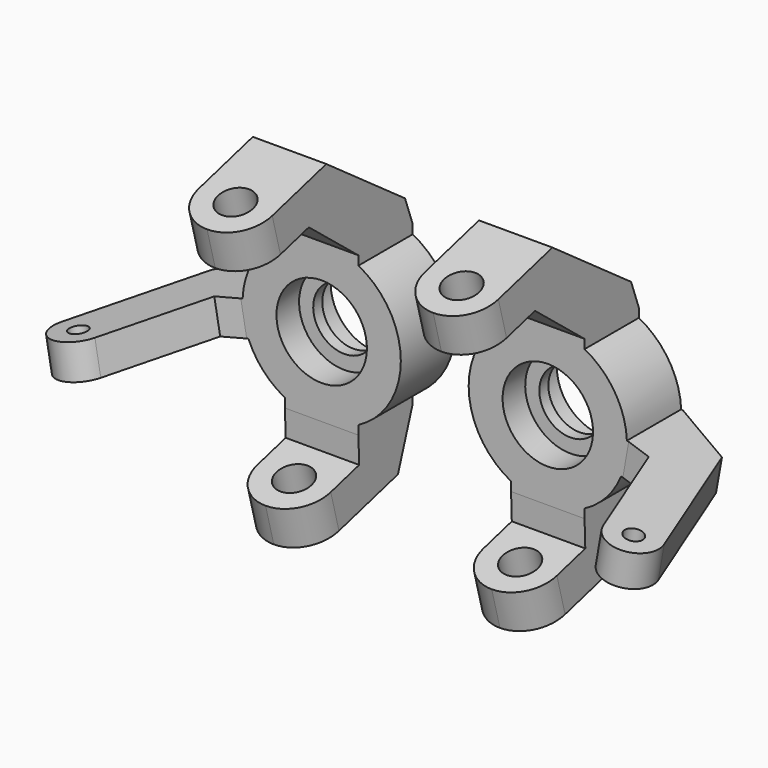
from build123d import *

# Parameters (mm, degrees)
F0_R      = 14
F1_DEPTH  = 12
F3_DEPTH  = 6.5
F4_R      = 6.49999
F5_R      = 3.1
F6_DEPTH  = 61.7194243546
F9_R      = 1.6
F10_DEPTH = 3


# Not quite as in the source:
# - a fillet or chamfer is up to 0.001 mm smaller than in the source, because OpenCascade refuses the exact size


with BuildPart() as f1:
    # F0 (on Front) → F1 (new body)
    with BuildSketch(Plane.XZ):
        Circle(F0_R)
    extrude(amount=F1_DEPTH)

    # F2 (on Right) → F3 (join, symmetric)
    with BuildSketch(Plane.YZ):
        Polygon((-37.3368032832, 26.2287753615), (-35.5250699675, 19.4672945775), (-22.9680342257, 22.8319421638), (-12, 14), (-12, -14), (-11.8388152863, -18.7028683666), (-24.3958510281, -22.0675159529), (-22.5841177123, -28.828996737), (-3.2656011866, -23.6526158349), (0, -14), (0, 14), (-1.7101007166, 18.6984631039), (-19.1062115093, 31.1136477049), align=None)
    extrude(amount=F3_DEPTH, both=True)

    # F4 (radius 6.5 in the source; OpenCascade refuses exactly that, so slightly less here)
    f4_edges = [f1.edges().sort_by_distance(p)[0] for p in [
        (-6.5, -36.430937, 22.848035),
        (6.5, -36.430937, 22.848035),
        (-6.5, -23.489984, -25.448256),
        (6.5, -23.489984, -25.448256),
    ]]
    fillet(f4_edges, radius=F4_R)

    # F5 (on face) → F6 (cut, through all)
    with BuildSketch(Plane(origin=(0, 5.6944001585, -21.2517907103), x_dir=(1, 0, 0), z_dir=(0, 0.2588190451, -0.9659258263))):
        with Locations((0, 22.776075969)):
            Circle(F5_R)
    extrude(amount=-F6_DEPTH, mode=Mode.SUBTRACT)

    # F9 (on line) → F10 (join, symmetric)
    with BuildSketch(Plane(origin=(0, 0, 0), x_dir=(0.984807753, 0, 0.1736481777), z_dir=(0.1736481777, 0, -0.984807753))):
        with BuildLine():
            Line((-18.1775185709, 12.7166448356), (-24.8133673259, 30.9484894489))
            ThreePointArc((-24.8133673259, 30.9484894489), (-30.5810747644, 33.6380155974), (-33.270600913, 27.8703081589))
            Line((-33.270600913, 27.8703081589), (-24.8575633616, 4.7556774576))
            Line((-24.8575633616, 4.7556774576), (-14, 0))
            Line((-14, 0), (-3.9701759072, 0))
            Line((-3.9701759072, 0), (-3.9701759072, 12))
            Line((-3.9701759072, 12), (-14, 12))
            Line((-14, 12), (-18.1775185709, 12.7166448356))
        make_face()
        with Locations((-29.0419841195, 29.4093988039)):
            Circle(F9_R, mode=Mode.SUBTRACT)
    extrude(amount=F10_DEPTH, both=True)

    # F11 (on Right) → F12 (revolve, cut)
    with BuildSketch(Plane.YZ):
        Polygon((0, 0), (0, 8), (-5, 8), (-5, 5.5), (-7, 5.5), (-7, 8), (-12, 8), (-12, 0), align=None)
    revolve(axis=Axis((0, 2.6090382598, 0), (0, 1, 0)), mode=Mode.SUBTRACT)


with BuildPart() as f14_1:
    # F14: instance of F1
    add(f1.part.mirror(Plane.YZ.offset(20)))


solid = Compound([f1.part, f14_1.part])
